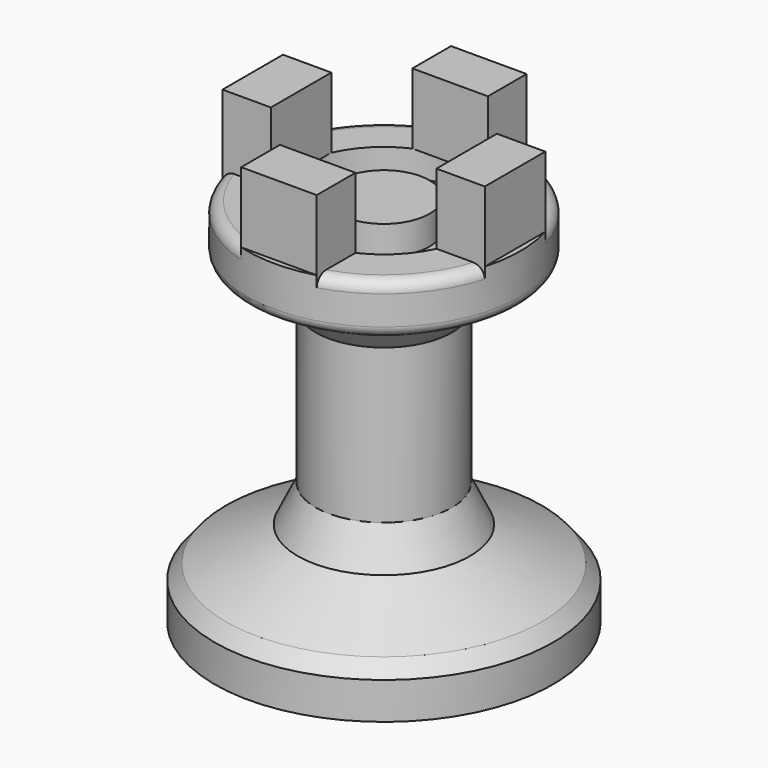
from build123d import *

# Parameters (mm, degrees)
F6_W         = 8.4365679183
F6_H         = 5.4016525666
F6_W_2       = 5.4016525666
F6_H_2       = 8.4365679183
F7_DEPTH     = 7.874
F8_T6_ANGLE  = 57.8625360508
F8_T12_ANGLE = 57.8625360508
F8_T18_ANGLE = 57.8625360508
F8_T24_ANGLE = 57.8625360508
F9_SIZE      = 5.08


# Not quite as in the source:
# - a fillet or chamfer that OpenCascade refuses, or shapes differently, is made with other operations: its cross-section is extruded or revolved along the edge and cut away or added


with BuildPart() as f1:
    # F0 (on Front) → F1 (revolve)
    with BuildSketch(Plane.XZ):
        Polygon((-18.9049374312, -5.9133931063), (0, -5.9133931063), (0, 3.7630684674), (-14.4250961021, 3.7630684674), (-18.9049374312, -1.7919373931), align=None)
    revolve(axis=Axis((0, 0, -1.0751623195), (0, 0, -1)))

    # F9
    f9_edges = [f1.edges().sort_by_distance(p)[0] for p in [
        (14.425096, 0, 3.763068),
    ]]
    chamfer(f9_edges, length=F9_SIZE)


with BuildPart() as f3:
    # F2 (on Front) → F3 (revolve)
    with BuildSketch(Plane.XZ):
        Polygon((-7.62, 7.8041334668), (-9.6175679059, 3.6735106291), (0, 3.6735106291), (0, 7.8041334668), align=None)
        Polygon((-7.62, 25.0067324409), (-7.62, 7.8041334668), (0, 7.8041334668), (0, 25.0643868962), (0, 29.0066474148), (-11.2038745534, 29.0066474148), align=None)
    revolve(axis=Axis((0, 0, 12.5321934481), (0, 0, -1)))


with BuildPart() as f5:
    # F4 (on Front) → F5 (revolve)
    with BuildSketch(Plane.XZ):
        Polygon((-15.24, 30.283741653), (-12.6989696556, 28.8676137807), (0, 29.0293842554), (0, 35.8387455344), (-5.08, 35.8387455344), (-5.08, 32.6132588089), (-10.16, 32.6132588089), (-10.16, 35.4803577065), (-15.24, 35.4803577065), align=None)
    revolve(axis=Axis((0, 0, 32.4340648949), (0, 0, -1)))

    # F6 (on face) → F7 (join)
    with BuildSketch(Plane.XY.offset(35.4803577065)):
        with Locations((0, 11.9437522508)):
            Rectangle(F6_W, F6_H)
        with Locations((11.9437522508, 0)):
            Rectangle(F6_W_2, F6_H_2)
        with Locations((-11.9437522508, 0)):
            Rectangle(F6_W_2, F6_H_2)
        with Locations((0, -11.9437522508)):
            Rectangle(F6_W, F6_H)
    extrude(amount=F7_DEPTH)

    # F8: fillet of radius 1.27 on 6 edges, made by hand

    # F8_s1 → F8_t2 (revolve, cut)
    with BuildSketch(Plane.XZ):
        with BuildLine():
            ThreePointArc((-14.587416998, 29.9195962274), (-15.0650751907, 30.3865108079), (-15.2404, 31.031047685))
            Line((-15.2404, 31.031047685), (-15.36764, 31.031047685))
            ThreePointArc((-15.36764, 31.031047685), (-15.36724, 30.657394669), (-15.36724, 30.283741653))
            Line((-15.36724, 30.283741653), (-15.3019416998, 30.1725965072))
            ThreePointArc((-15.3019416998, 30.1725965072), (-14.9755528368, 29.990698496), (-14.6493586978, 29.8084510816))
            Line((-14.6493586978, 29.8084510816), (-14.587416998, 29.9195962274))
        make_face()
    revolve(axis=Axis((0, 0, 30.283741653), (0, 0, -1)), mode=Mode.SUBTRACT)


with BuildPart() as f8_tool4:
    # F8_s5 → F8_t6 (revolve)
    with BuildSketch(Plane(origin=(0, 0, 0), x_dir=(0, 0, 1), z_dir=(0.96093035, -0.276790286, 0))):
        with BuildLine():
            ThreePointArc((34.2093920211, 15.2404), (35.1083833187, 14.8680256121), (35.4807577065, 13.9690343146))
            Line((35.4807577065, 13.9690343146), (35.6078942751, 13.9690343146))
            ThreePointArc((35.6078942751, 13.9690343146), (35.6074942751, 14.6045171573), (35.6074942751, 15.24))
            Line((35.6074942751, 15.24), (35.4803577065, 15.3671365685))
            ThreePointArc((35.4803577065, 15.3671365685), (34.8448748638, 15.3671365685), (34.2093920211, 15.3675365685))
            Line((34.2093920211, 15.3675365685), (34.2093920211, 15.2404))
        make_face()
    revolve(axis=Axis((0, 0, 35.4803577065), (0, 0, -1)), revolution_arc=F8_T6_ANGLE)

    split(bisect_by=Plane.YZ.offset(-4.2182839591), keep=Keep.BOTTOM)

    split(bisect_by=Plane.XZ.offset(4.2182839591), keep=Keep.TOP)


with BuildPart() as f5_1:
    add(f5.part)

    # F8_t3: cut F8_tool4
    add(f8_tool4.part, mode=Mode.SUBTRACT)


with BuildPart() as f8_tool10:
    # F8_s11 → F8_t12 (revolve)
    with BuildSketch(Plane(origin=(0, 0, 0), x_dir=(0, 0, 1), z_dir=(0.276790286, 0.96093035, 0))):
        with BuildLine():
            ThreePointArc((34.2093920211, 15.2404), (35.1083833187, 14.8680256121), (35.4807577065, 13.9690343146))
            Line((35.4807577065, 13.9690343146), (35.6078942751, 13.9690343146))
            ThreePointArc((35.6078942751, 13.9690343146), (35.6074942751, 14.6045171573), (35.6074942751, 15.24))
            Line((35.6074942751, 15.24), (35.4803577065, 15.3671365685))
            ThreePointArc((35.4803577065, 15.3671365685), (34.8448748638, 15.3671365685), (34.2093920211, 15.3675365685))
            Line((34.2093920211, 15.3675365685), (34.2093920211, 15.2404))
        make_face()
    revolve(axis=Axis((0, 0, 35.4803577065), (0, 0, -1)), revolution_arc=F8_T12_ANGLE)

    split(bisect_by=Plane.XZ.offset(4.2182839591), keep=Keep.TOP)

    split(bisect_by=Plane.YZ.offset(4.2182839591), keep=Keep.TOP)


with BuildPart() as f5_2:
    add(f5_1.part)

    # F8_t9: cut F8_tool10
    add(f8_tool10.part, mode=Mode.SUBTRACT)


with BuildPart() as f8_tool16:
    # F8_s17 → F8_t18 (revolve)
    with BuildSketch(Plane(origin=(0, 0, 0), x_dir=(0, 0, 1), z_dir=(-0.96093035, 0.276790286, 0))):
        with BuildLine():
            ThreePointArc((34.2093920211, 15.2404), (35.1083833187, 14.8680256121), (35.4807577065, 13.9690343146))
            Line((35.4807577065, 13.9690343146), (35.6078942751, 13.9690343146))
            ThreePointArc((35.6078942751, 13.9690343146), (35.6074942751, 14.6045171573), (35.6074942751, 15.24))
            Line((35.6074942751, 15.24), (35.4803577065, 15.3671365685))
            ThreePointArc((35.4803577065, 15.3671365685), (34.8448748638, 15.3671365685), (34.2093920211, 15.3675365685))
            Line((34.2093920211, 15.3675365685), (34.2093920211, 15.2404))
        make_face()
    revolve(axis=Axis((0, 0, 35.4803577065), (0, 0, -1)), revolution_arc=F8_T18_ANGLE)

    split(bisect_by=Plane.YZ.offset(4.2182839591), keep=Keep.TOP)

    split(bisect_by=Plane.XZ.offset(-4.2182839591), keep=Keep.BOTTOM)


with BuildPart() as f5_3:
    add(f5_2.part)

    # F8_t15: cut F8_tool16
    add(f8_tool16.part, mode=Mode.SUBTRACT)


with BuildPart() as f8_tool22:
    # F8_s23 → F8_t24 (revolve)
    with BuildSketch(Plane(origin=(0, 0, 0), x_dir=(0, 0, 1), z_dir=(-0.276790286, -0.96093035, 0))):
        with BuildLine():
            ThreePointArc((34.2093920211, 15.2404), (35.1083833187, 14.8680256121), (35.4807577065, 13.9690343146))
            Line((35.4807577065, 13.9690343146), (35.6078942751, 13.9690343146))
            ThreePointArc((35.6078942751, 13.9690343146), (35.6074942751, 14.6045171573), (35.6074942751, 15.24))
            Line((35.6074942751, 15.24), (35.4803577065, 15.3671365685))
            ThreePointArc((35.4803577065, 15.3671365685), (34.8448748638, 15.3671365685), (34.2093920211, 15.3675365685))
            Line((34.2093920211, 15.3675365685), (34.2093920211, 15.2404))
        make_face()
    revolve(axis=Axis((0, 0, 35.4803577065), (0, 0, -1)), revolution_arc=F8_T24_ANGLE)

    split(bisect_by=Plane.XZ.offset(-4.2182839591), keep=Keep.BOTTOM)

    split(bisect_by=Plane.YZ.offset(-4.2182839591), keep=Keep.BOTTOM)


with BuildPart() as f5_4:
    add(f5_3.part)

    # F8_t21: cut F8_tool22
    add(f8_tool22.part, mode=Mode.SUBTRACT)


solid = Compound([f1.part, f3.part, f5_4.part])
